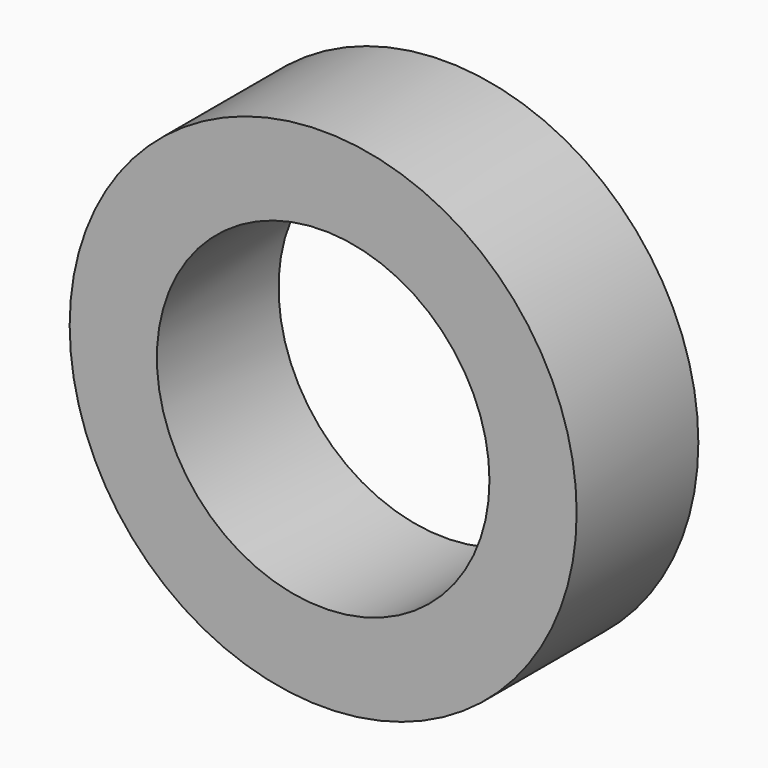
from build123d import *

# Parameters (mm, degrees)
F0_R     = 3.96875
F0_R_2   = 2.6035
F1_DEPTH = 2.38125


# Not quite as in the source:
# - a length typed as a fraction of an inch, garbled in the dataset ("3 / 203.2 mm" for 3/8 in), is restored


with BuildPart() as f1:
    # F0 (on Front) → F1 (new body)
    with BuildSketch(Plane.XZ):
        Circle(F0_R)
        Circle(F0_R_2, mode=Mode.SUBTRACT)
    extrude(amount=F1_DEPTH)


solid = f1.part
